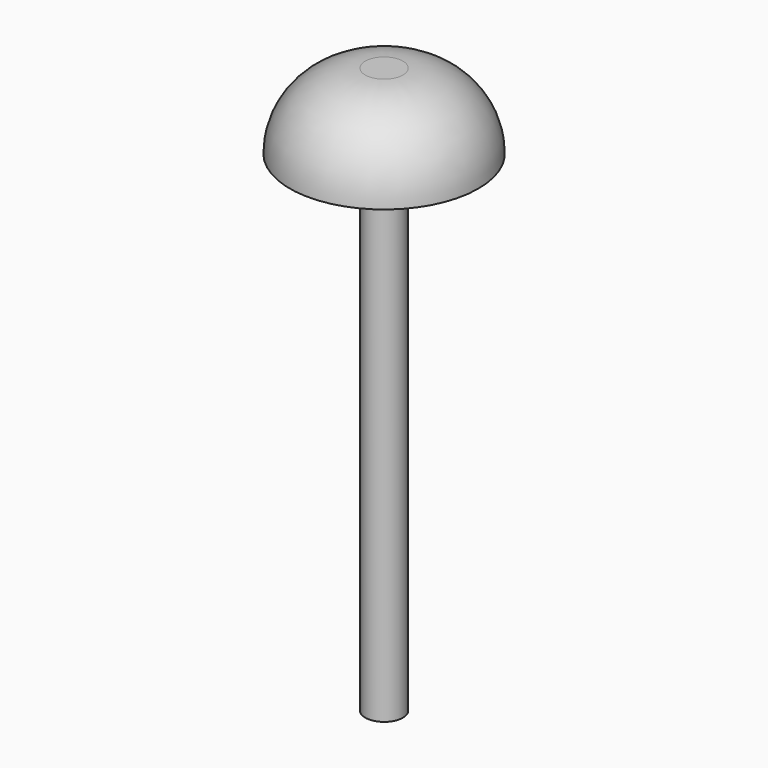
from build123d import *

# Parameters (mm, degrees)
F0_R     = 1.27
F1_DEPTH = 33.02
F2_R     = 6.35
F3_DEPTH = 5.08
F4_R     = 5.07999


# Not quite as in the source:
# - a fillet or chamfer is up to 0.001 mm smaller than in the source, because OpenCascade refuses the exact size


with BuildPart() as f1:
    # F0 (on Top) → F1 (new body)
    with BuildSketch(Plane.XY):
        Circle(F0_R)
    extrude(amount=F1_DEPTH)

    # F2 (on face) → F3 (join)
    with BuildSketch(Plane.XY.offset(33.02)):
        Circle(F2_R)
    extrude(amount=F3_DEPTH)

    # F4 (radius 5.08 in the source; OpenCascade refuses exactly that, so slightly less here)
    f4_edges = [f1.edges().sort_by_distance(p)[0] for p in [
        (-6.35, 0, 38.1),
    ]]
    fillet(f4_edges, radius=F4_R)


solid = f1.part
